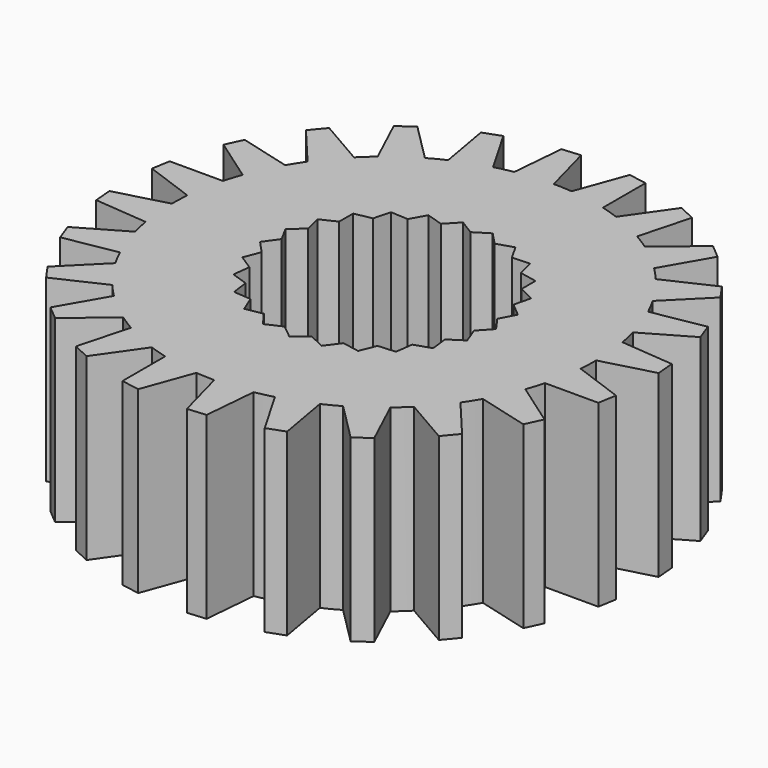
from build123d import *

# Parameters (mm, degrees)
F1_DEPTH = 5.08


# Not quite as in the source:
# - ends of sketch curves that miss each other by under 0.0002 mm in the source are joined


with BuildPart() as f1:
    # F0 (on Top) → F1 (new body)
    with BuildSketch(Plane.XY):
        with BuildLine():
            Line((1.0386822, 7.3975722), (0.5233416, 5.9817))
            ThreePointArc((0.5233416, 5.9817), (0.261920534, 5.9988447577), (0, 6.00456))
            Line((0, 6.00456), (-0.3899662, 7.4599546))
            Line((-0.3899662, 7.4599546), (-0.911352, 7.4143362))
            Line((-0.911352, 7.4143362), (-1.04267, 5.9133486))
            ThreePointArc((-1.04267, 5.9133486), (-1.2996201412, 5.8622289517), (-1.5540978425, 5.79995868))
            Line((-1.5540978425, 5.79995868), (-2.307463, 7.1048372))
            Line((-2.307463, 7.1048372), (-2.7992832, 6.925818))
            Line((-2.7992832, 6.925818), (-2.5376378, 5.4419754))
            ThreePointArc((-2.5376378, 5.4419754), (-2.7726007409, 5.3261079528), (-3.0022844594, 5.2000989239))
            Line((-3.0022844594, 5.2000989239), (-4.0677084, 6.2655196))
            Line((-4.0677084, 6.2655196), (-4.496435, 5.965317))
            Line((-4.496435, 5.965317), (-3.859657, 4.5997622))
            ThreePointArc((-3.859657, 4.5997622), (-4.0566214385, 4.4270264624), (-4.245865094, 4.245865094))
            Line((-4.245865094, 4.245865094), (-5.5507382, 4.999228))
            Line((-5.5507382, 4.999228), (-5.8871612, 4.598289))
            Line((-5.8871612, 4.598289), (-4.9186338, 3.4440622))
            ThreePointArc((-4.9186338, 3.4440622), (-5.0641936548, 3.2262491255), (-5.2000989239, 3.0022844594))
            Line((-5.2000989239, 3.0022844594), (-6.6554858, 3.3922462))
            Line((-6.6554858, 3.3922462), (-6.876669, 2.9179012))
            Line((-6.876669, 2.9179012), (-5.6424322, 2.0536916))
            ThreePointArc((-5.6424322, 2.0536916), (-5.7266481207, 1.8056140494), (-5.79995868, 1.5540978425))
            Line((-5.79995868, 1.5540978425), (-7.306691, 1.554099))
            Line((-7.306691, 1.554099), (-7.3975722, 1.0386568))
            Line((-7.3975722, 1.0386568), (-5.9817, 0.5233416))
            ThreePointArc((-5.9817, 0.5233416), (-5.9988447577, 0.261920534), (-6.00456, 0))
            Line((-6.00456, 0), (-7.4599546, -0.3899662))
            Line((-7.4599546, -0.3899662), (-7.4143362, -0.911352))
            Line((-7.4143362, -0.911352), (-5.9133232, -1.04267))
            ThreePointArc((-5.9133232, -1.04267), (-5.8622284744, -1.2996222942), (-5.79995868, -1.5540978425))
            Line((-5.79995868, -1.5540978425), (-7.1048372, -2.307463))
            Line((-7.1048372, -2.307463), (-6.925818, -2.7992832))
            Line((-6.925818, -2.7992832), (-5.4419754, -2.5376378))
            ThreePointArc((-5.4419754, -2.5376378), (-5.3261079528, -2.7726007409), (-5.2000989239, -3.0022844594))
            Line((-5.2000989239, -3.0022844594), (-6.2655196, -4.0677084))
            Line((-6.2655196, -4.0677084), (-5.965317, -4.496435))
            Line((-5.965317, -4.496435), (-4.5997622, -3.859657))
            ThreePointArc((-4.5997622, -3.859657), (-4.4270264624, -4.0566214385), (-4.245865094, -4.245865094))
            Line((-4.245865094, -4.245865094), (-4.999228, -5.5507382))
            Line((-4.999228, -5.5507382), (-4.598289, -5.8871612))
            Line((-4.598289, -5.8871612), (-3.4440622, -4.9186592))
            ThreePointArc((-3.4440622, -4.9186592), (-3.2262429819, -5.0641975688), (-3.0022844594, -5.2000989239))
            Line((-3.0022844594, -5.2000989239), (-3.3922462, -6.6554858))
            Line((-3.3922462, -6.6554858), (-2.9179012, -6.8766944))
            Line((-2.9179012, -6.8766944), (-2.0536662, -5.6424322))
            ThreePointArc((-2.0536662, -5.6424322), (-1.8056026676, -5.7266517094), (-1.5540978425, -5.79995868))
            Line((-1.5540978425, -5.79995868), (-1.554099, -7.306691))
            Line((-1.554099, -7.306691), (-1.0386568, -7.3975722))
            Line((-1.0386568, -7.3975722), (-0.5233162, -5.9817))
            ThreePointArc((-0.5233162, -5.9817), (-0.2619078943, -5.9988453096), (0, -6.00456))
            Line((0, -6.00456), (0.3899662, -7.4599546))
            Line((0.3899662, -7.4599546), (0.9113774, -7.4143362))
            Line((0.9113774, -7.4143362), (1.0426954, -5.9133486))
            ThreePointArc((1.0426954, -5.9133486), (1.2996323518, -5.8622262447), (1.5540978425, -5.79995868))
            Line((1.5540978425, -5.79995868), (2.307463, -7.1048372))
            Line((2.307463, -7.1048372), (2.7992832, -6.925818))
            Line((2.7992832, -6.925818), (2.5376378, -5.4419754))
            ThreePointArc((2.5376378, -5.4419754), (2.7726007409, -5.3261079528), (3.0022844594, -5.2000989239))
            Line((3.0022844594, -5.2000989239), (4.0677084, -6.2655196))
            Line((4.0677084, -6.2655196), (4.496435, -5.965317))
            Line((4.496435, -5.965317), (3.859657, -4.5997622))
            ThreePointArc((3.859657, -4.5997622), (4.0566214385, -4.4270264624), (4.245865094, -4.245865094))
            Line((4.245865094, -4.245865094), (5.5507382, -4.999228))
            Line((5.5507382, -4.999228), (5.8871612, -4.598289))
            Line((5.8871612, -4.598289), (4.9186592, -3.4440622))
            ThreePointArc((4.9186592, -3.4440622), (5.0642009806, -3.2262376264), (5.2001052739, -3.0022734609))
            Line((5.2001052739, -3.0022734609), (6.6555112, -3.3922462))
            Line((6.6555112, -3.3922462), (6.8766944, -2.9179012))
            Line((6.8766944, -2.9179012), (5.6424576, -2.0536916))
            ThreePointArc((5.6424576, -2.0536916), (5.7266494269, -1.8056099067), (5.79995868, -1.5540978425))
            Line((5.79995868, -1.5540978425), (7.306691, -1.554099))
            Line((7.306691, -1.554099), (7.3975722, -1.0386568))
            Line((7.3975722, -1.0386568), (5.9817254, -0.5233416))
            ThreePointArc((5.9817254, -0.5233416), (5.998844806, -0.2619194281), (6.00456, 0))
            Line((6.00456, 0), (7.4599546, 0.3899662))
            Line((7.4599546, 0.3899662), (7.4143362, 0.911352))
            Line((7.4143362, 0.911352), (5.9133486, 1.04267))
            ThreePointArc((5.9133486, 1.04267), (5.8622289517, 1.2996201412), (5.79995868, 1.5540978425))
            Line((5.79995868, 1.5540978425), (7.1048372, 2.307463))
            Line((7.1048372, 2.307463), (6.925818, 2.7992832))
            Line((6.925818, 2.7992832), (5.4419754, 2.5376378))
            ThreePointArc((5.4419754, 2.5376378), (5.3261108849, 2.7725951084), (5.2001052739, 3.0022734609))
            Line((5.2001052739, 3.0022734609), (6.2655196, 4.0677084))
            Line((6.2655196, 4.0677084), (5.9653424, 4.496435))
            Line((5.9653424, 4.496435), (4.5997622, 3.859657))
            ThreePointArc((4.5997622, 3.859657), (4.4270264624, 4.0566214385), (4.245865094, 4.245865094))
            Line((4.245865094, 4.245865094), (4.999228, 5.5507382))
            Line((4.999228, 5.5507382), (4.5983144, 5.8871612))
            Line((4.5983144, 5.8871612), (3.4440876, 4.9186592))
            ThreePointArc((3.4440876, 4.9186592), (3.2262517559, 5.0641919791), (3.0022844594, 5.2000989239))
            Line((3.0022844594, 5.2000989239), (3.3922462, 6.6554858))
            Line((3.3922462, 6.6554858), (2.9179012, 6.8766944))
            Line((2.9179012, 6.8766944), (2.0536916, 5.6424322))
            ThreePointArc((2.0536916, 5.6424322), (1.8056140494, 5.7266481207), (1.5540978425, 5.79995868))
            Line((1.5540978425, 5.79995868), (1.554099, 7.306691))
            Line((1.554099, 7.306691), (1.0386822, 7.3975722))
        make_face()
        Polygon((-1.2318492, 3.1113222), (-0.7605522, 2.9622242), (-0.4194048, 3.319907), (0, 3.0583124), (0.4194048, 3.319907), (0.7605776, 2.9622242), (1.2318492, 3.1113222), (1.4733524, 2.6800048), (1.9668998, 2.7072082), (2.0935442, 2.2294088), (2.5783794, 2.1330158), (2.5822148, 1.6387318), (3.0278324, 1.4247876), (2.9086302, 0.9450578), (3.2870394, 0.6270244), (3.0522672, 0.192024), (3.3396936, -0.2101088), (3.0041342, -0.5730748), (3.1825184, -1.0340594), (2.7672284, -1.3021564), (2.825369, -1.7930368), (2.3564596, -1.9494246), (2.290699, -2.4393398), (1.7976342, -2.474214), (1.6120872, -2.9323792), (1.1258296, -2.84353), (0.8322056, -3.241167), (0.3833114, -3.0341824), (0, -3.3462976), (-0.3833114, -3.0341824), (-0.8321802, -3.241167), (-1.1258296, -2.84353), (-1.6120872, -2.9323792), (-1.7976088, -2.474214), (-2.290699, -2.4393398), (-2.3564596, -1.9494246), (-2.825369, -1.7930368), (-2.7672284, -1.3021564), (-3.1825184, -1.0340594), (-3.0041342, -0.5730748), (-3.3396936, -0.2101088), (-3.0522672, 0.192024), (-3.287014, 0.6270244), (-2.9086048, 0.9450578), (-3.027807, 1.4247876), (-2.5822148, 1.6387318), (-2.578354, 2.1330158), (-2.0935442, 2.2294088), (-1.9668998, 2.7072082), (-1.4733524, 2.6800048), align=None, mode=Mode.SUBTRACT)
    extrude(amount=F1_DEPTH)


solid = f1.part
